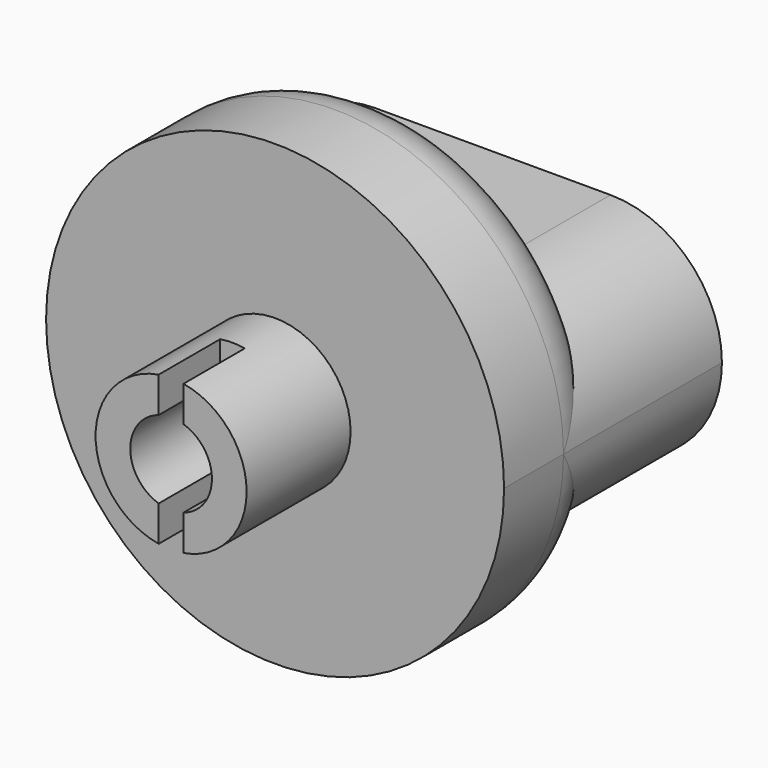
from build123d import *

# Parameters (mm, degrees)
F0_R      = 6.1
F0_R_2    = 3.3
F1_DEPTH  = 20
F4_DEPTH  = 2
F6_W      = 37
F6_H      = 18
F7_DEPTH  = 22
F8_R      = 8.99999
F9_R      = 8.99999
F10_R     = 8.99999
F12_W     = 2
F12_H     = 13
F13_DEPTH = 8.2
F14_R     = 3.3
F15_DEPTH = 10
F17_DEPTH = 2


# Not quite as in the source:
# - a fillet or chamfer is up to 0.001 mm smaller than in the source, because OpenCascade refuses the exact size


with BuildPart() as f1:
    # F0 (on Front) → F1 (new body)
    with BuildSketch(Plane.XZ):
        Circle(F0_R)
        Circle(F0_R_2, mode=Mode.SUBTRACT)
    extrude(amount=-F1_DEPTH)

    # F2 (on Top) → F3 (revolve)
    with BuildSketch(Plane.XY):
        with BuildLine():
            Line((-18.5, 12.5), (0, 12.5))
            Line((0, 12.5), (0, 23.5))
            Line((0, 23.5), (-13.5, 23.5))
            ThreePointArc((-13.5, 23.5), (-17.0355339059, 22.0355339059), (-18.5, 18.5))
            Line((-18.5, 18.5), (-18.5, 12.5))
        make_face()
    revolve(axis=Axis((0, 18, 0), (0, 1, 0)))

    # F0 (on Front) → F4 (cut)
    with BuildSketch(Plane.XZ):
        Circle(F0_R)
        Circle(F0_R_2, mode=Mode.SUBTRACT)
    extrude(amount=-F4_DEPTH, mode=Mode.SUBTRACT)

    # F6 (on offset) → F7 (join)
    with BuildSketch(Plane.XZ.offset(-12.5)):
        Rectangle(F6_W, F6_H)
    extrude(amount=-F7_DEPTH)

    # F8 (radius 9 in the source; OpenCascade refuses exactly that, so slightly less here)
    f8_edges = [f1.edges().sort_by_distance(p)[0] for p in [
        (-18.5, 23.5, -9),
    ]]
    fillet(f8_edges, radius=F8_R)

    # F9 (radius 9 in the source; OpenCascade refuses exactly that, so slightly less here)
    f9_edges = [f1.edges().sort_by_distance(p)[0] for p in [
        (-18.5, 23.5, 9),
    ]]
    fillet(f9_edges, radius=F9_R)

    # F10 (radius 9 in the source; OpenCascade refuses exactly that, so slightly less here)
    f10_edges = [f1.edges().sort_by_distance(p)[0] for p in [
        (18.5, 23.5, -9),
        (18.5, 23.5, 9),
    ]]
    fillet(f10_edges, radius=F10_R)

    # F12 (on face) → F13 (cut)
    with BuildSketch(Plane.XZ):
        Rectangle(F12_W, F12_H)
    extrude(amount=-F13_DEPTH, mode=Mode.SUBTRACT)

    # F14 (on face) → F15 (cut)
    with BuildSketch(Plane.XZ.offset(-12.5)):
        Circle(F14_R)
    extrude(amount=-F15_DEPTH, mode=Mode.SUBTRACT)

    # F16 (on offset) → F17 (cut)
    with BuildSketch(Plane(origin=(0, 34.5, 0), x_dir=(-1, 0, 0), z_dir=(0, 1, 0))):
        with BuildLine():
            ThreePointArc((16, -1), (17, 0), (16, 1))
            Line((16, 1), (9, 1))
            ThreePointArc((9, 1), (8, 0), (9, -1))
            Line((9, -1), (16, -1))
        make_face()
    extrude(amount=-F17_DEPTH, mode=Mode.SUBTRACT)


solid = f1.part
